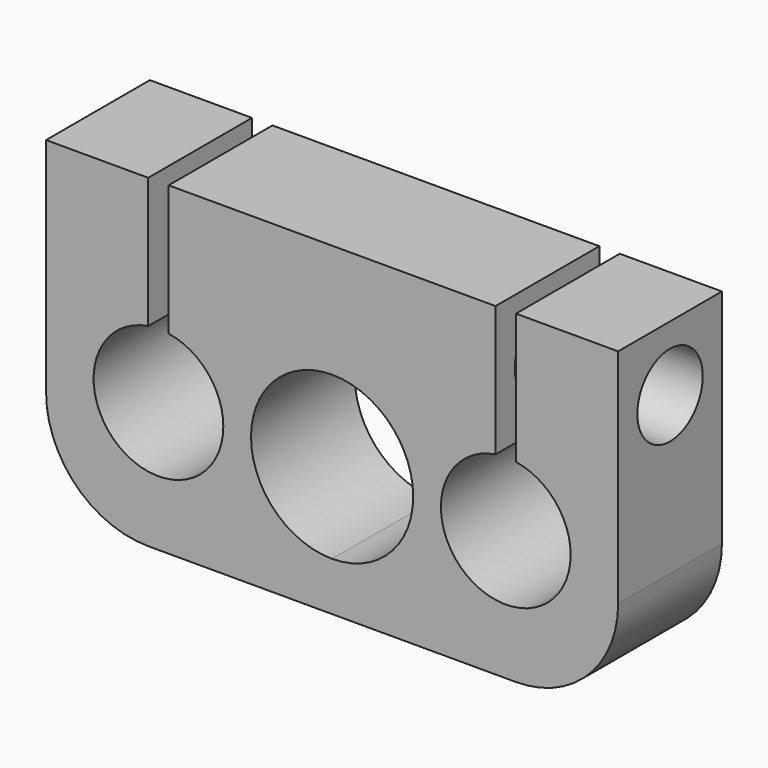
from build123d import *

# Parameters (mm, degrees)
F1_DEPTH = 6.35
F2_R     = 2
F3_DEPTH = 22.5
F4_R     = 5
F5_R     = 1.75
F6_DEPTH = 28.001


# Not quite as in the source:
# - a feature names something its author has since deleted; it is built from what else it names


with BuildPart() as f1:
    # F0 (on Front) → F1 (new body)
    with BuildSketch(Plane.XZ):
        with BuildLine():
            ThreePointArc((0, -3.96875), (-3.96875, 0), (0, 3.96875))
            Line((0, 3.96875), (0, 9.525))
            Line((0, 9.525), (-8, 9.525))
            Line((-8, 9.525), (-8, 3.1353827518))
            ThreePointArc((-8, 3.1353827518), (-6.0846195952, 2.0607189279), (-5.325, 0))
            ThreePointArc((-5.325, 0), (-10.5607189279, -2.4153804048), (-9, 3.1353827518))
            Line((-9, 3.1353827518), (-9, 9.525))
            Line((-9, 9.525), (-14, 9.525))
            Line((-14, 9.525), (-14, -6.35))
            Line((-14, -6.35), (0, -6.35))
            Line((0, -6.35), (0, -3.96875))
        make_face()
        with BuildLine():
            ThreePointArc((0, 3.96875), (2.8063300378, 2.8063300378), (3.96875, 0))
            ThreePointArc((3.96875, 0), (2.8063300378, -2.8063300378), (0, -3.96875))
            Line((0, -3.96875), (0, -6.35))
            Line((0, -6.35), (14, -6.35))
            Line((14, -6.35), (14, 9.525))
            Line((14, 9.525), (9, 9.525))
            Line((9, 9.525), (9, 3.1353827518))
            ThreePointArc((9, 3.1353827518), (10.9153804048, 2.0607189279), (11.675, 0))
            ThreePointArc((11.675, 0), (6.4392810721, -2.4153804048), (8, 3.1353827518))
            Line((8, 3.1353827518), (8, 9.525))
            Line((8, 9.525), (0, 9.525))
            Line((0, 9.525), (0, 3.96875))
        make_face()
    extrude(amount=F1_DEPTH)

    # F2 (on face) → F3 (cut)
    with BuildSketch(Plane.YZ.offset(14)):
        with Locations((-3.175, 6.35)):
            Circle(F2_R)
    extrude(amount=-F3_DEPTH, mode=Mode.SUBTRACT)

    # F4
    f4_edges = [f1.edges().sort_by_distance(p)[0] for p in [
        (14, -3.175, -6.35),
        (-14, -3.175, -6.35),
    ]]
    fillet(f4_edges, radius=F4_R)

    # F5 (on face) → F6 (cut, through all)
    with BuildSketch(Plane(origin=(-14, 0, 0), x_dir=(0, -1, 0), z_dir=(-1, 0, 0))):
        with Locations((3.175, 6.35)):
            Circle(F5_R)
    extrude(amount=-F6_DEPTH, mode=Mode.SUBTRACT)


solid = f1.part
